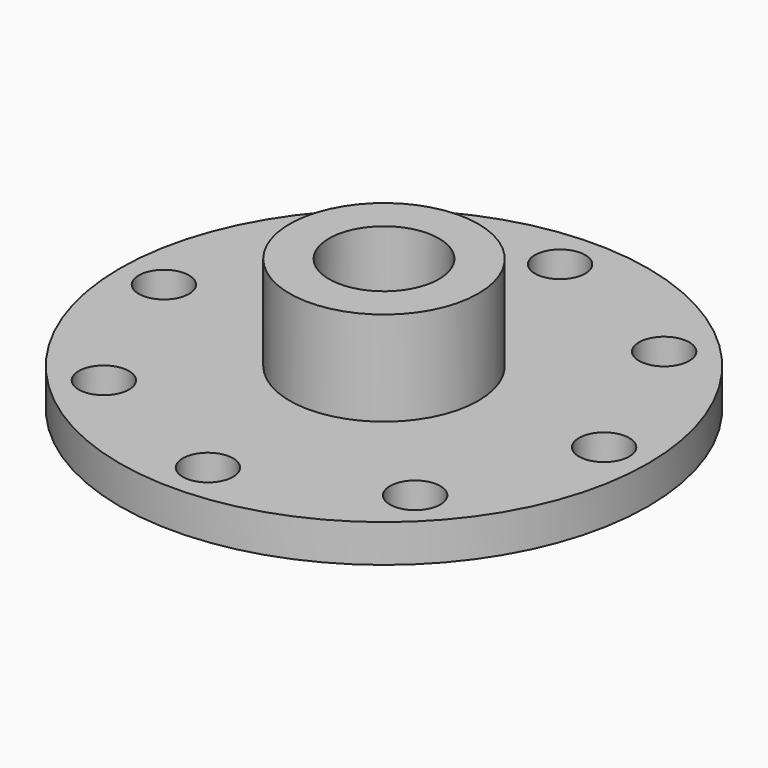
from build123d import *

# Parameters (mm, degrees)
F0_R     = 15
F0_R_2   = 8.75
F1_DEPTH = 21
F0_R_3   = 20
F2_DEPTH = 3
F0_R_4   = 42
F0_R_5   = 4
F3_DEPTH = 6
F4_DEPTH = 6
F0_R_6   = 5
F5_DEPTH = 3
F6_DEPTH = 3
F7_DEPTH = 1
F8_SIZE  = 3.74999


# Not quite as in the source:
# - a fillet or chamfer is up to 0.001 mm smaller than in the source, because OpenCascade refuses the exact size


with BuildPart() as f1:
    # F0 (on Top) → F1 (new body)
    with BuildSketch(Plane.XY):
        Circle(F0_R)
        Circle(F0_R_2, mode=Mode.SUBTRACT)
    extrude(amount=F1_DEPTH)

    # F0 (on Top) → F2 (join)
    with BuildSketch(Plane.XY):
        Circle(F0_R_3)
        Circle(F0_R, mode=Mode.SUBTRACT)
    extrude(amount=-F2_DEPTH)

    # F0 (on Top) → F3 (join)
    with BuildSketch(Plane.XY):
        Circle(F0_R_4)
        with Locations((-24.7487373415, -24.7487373415)):
            Circle(F0_R_5, mode=Mode.SUBTRACT)
        with Locations((0, -35)):
            Circle(F0_R_5, mode=Mode.SUBTRACT)
        with Locations((24.7487373415, -24.7487373415)):
            Circle(F0_R_5, mode=Mode.SUBTRACT)
        with Locations((-35, 0)):
            Circle(F0_R_5, mode=Mode.SUBTRACT)
        with Locations((-24.7487373415, 24.7487373415)):
            Circle(F0_R_5, mode=Mode.SUBTRACT)
        Circle(F0_R_3, mode=Mode.SUBTRACT)
        with Locations((35, 0)):
            Circle(F0_R_5, mode=Mode.SUBTRACT)
        with Locations((0, 35)):
            Circle(F0_R_5, mode=Mode.SUBTRACT)
        with Locations((24.7487373415, 24.7487373415)):
            Circle(F0_R_5, mode=Mode.SUBTRACT)
    extrude(amount=F3_DEPTH)

    # F0 (on Top) → F4 (join)
    with BuildSketch(Plane.XY):
        Circle(F0_R_3)
        Circle(F0_R, mode=Mode.SUBTRACT)
    extrude(amount=F4_DEPTH)

    # F0 (on Top) → F5 (join)
    with BuildSketch(Plane.XY):
        Circle(F0_R_2)
        Circle(F0_R_6, mode=Mode.SUBTRACT)
    extrude(amount=-F5_DEPTH)

    # F0 (on Top) → F6 (join)
    with BuildSketch(Plane.XY):
        Circle(F0_R)
        Circle(F0_R_2, mode=Mode.SUBTRACT)
    extrude(amount=-F6_DEPTH)

    # F0 (on Top) → F7 (join)
    with BuildSketch(Plane.XY):
        Circle(F0_R_2)
        Circle(F0_R_6, mode=Mode.SUBTRACT)
    extrude(amount=F7_DEPTH)

    # F8 (size 3.75 in the source; OpenCascade refuses exactly that, so slightly less here)
    f8_edges = [f1.edges().sort_by_distance(p)[0] for p in [
        (-8.75, 0, 1),
    ]]
    chamfer(f8_edges, length=F8_SIZE)


solid = f1.part
